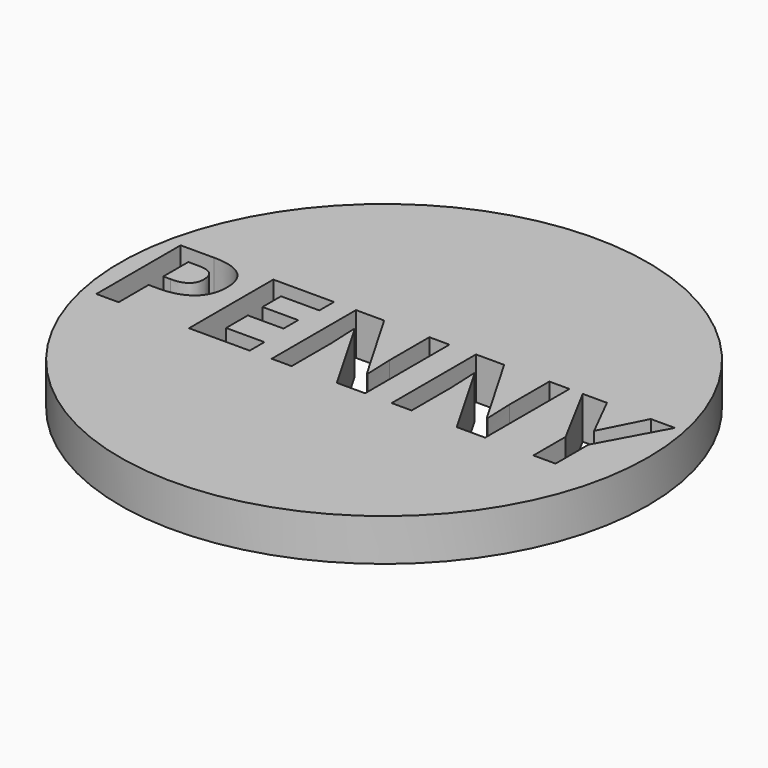
from build123d import *

# Parameters (mm, degrees)
F0_R         = 9.525
F1_DEPTH     = 1.52
F2_TEXT_SIZE = 5.3271146787
F3_DEPTH     = 25


# Not quite as in the source:
# - Text() gives the source's letters only with a copy of the font that has no kerning and outlines rounded to 1/6400 em; it was checked with that copy


with BuildPart() as f1:
    # F0 (on Top) → F1 (new body)
    with BuildSketch(Plane.XY):
        Circle(F0_R)
    extrude(amount=F1_DEPTH)

    # F2 (on face) → F3 (cut)
    with BuildSketch(Plane.XY.offset(1.52)):
        with Locations((-9.3299419428, -1.9177612843)):
            Text('PENNY', F2_TEXT_SIZE, font='Open Sans', font_style=FontStyle.BOLD, text_align=(TextAlign.LEFT, TextAlign.BOTTOM))
    extrude(amount=-F3_DEPTH, mode=Mode.SUBTRACT)


solid = f1.part
